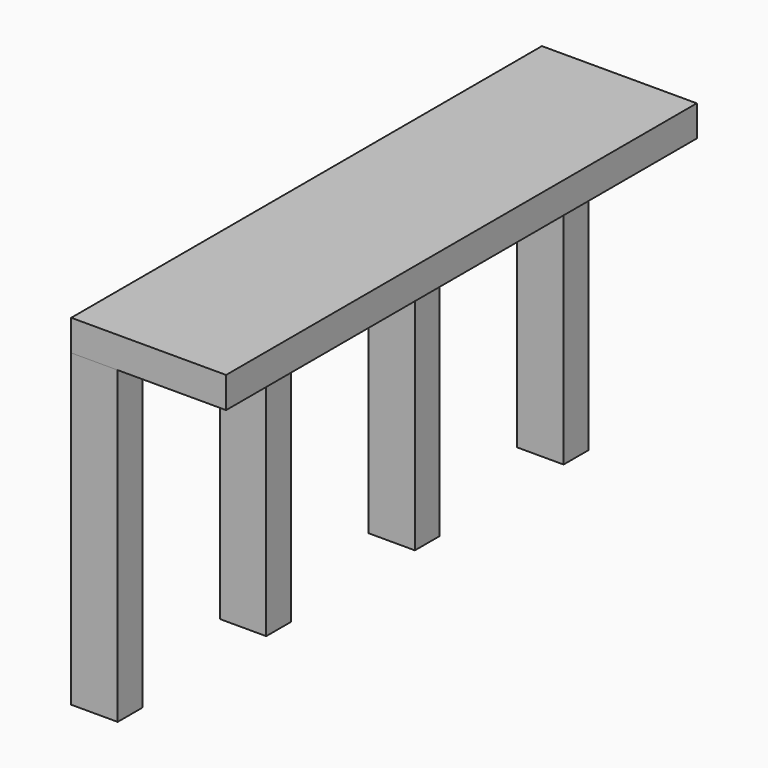
from build123d import *

# Parameters (mm, degrees)
F0_W     = 3
F0_H     = 2
F1_DEPTH = 20
F2_W     = 3
F2_H     = 2
F3_DEPTH = 2
F4_W     = 7.0251794532
F4_H     = 3.7774270773
F5_DEPTH = 25
F6_W     = 12.01007846
F6_H     = 2
F7_DEPTH = 25


with BuildPart() as f1:
    # F0 (on Top) → F1 (new body)
    with BuildSketch(Plane.XY):
        with Locations((1.5, 1)):
            Rectangle(F0_W, F0_H)
    extrude(amount=F1_DEPTH)


with BuildPart() as f1b:
    # F0 (on Top) → F1, piece 2 (new body)
    with BuildSketch(Plane.XY):
        with Locations((1.5, -11)):
            Rectangle(F0_W, F0_H)
    extrude(amount=F1_DEPTH)


with BuildPart() as f1c:
    # F0 (on Top) → F1, piece 3 (new body)
    with BuildSketch(Plane.XY):
        with Locations((1.5, -23)):
            Rectangle(F0_W, F0_H)
    extrude(amount=F1_DEPTH)


with BuildPart() as f1d:
    # F0 (on Top) → F1, piece 4 (new body)
    with BuildSketch(Plane.XY):
        with Locations((1.5, -35)):
            Rectangle(F0_W, F0_H)
    extrude(amount=F1_DEPTH)


with BuildPart() as f1e:
    # F0 (on Top) → F1, piece 5 (new body)
    with BuildSketch(Plane.XY):
        with Locations((1.5, -47)):
            Rectangle(F0_W, F0_H)
    extrude(amount=F1_DEPTH)


with BuildPart() as f1f:
    # F0 (on Top) → F1, piece 6 (new body)
    with BuildSketch(Plane.XY):
        with Locations((1.5, -59)):
            Rectangle(F0_W, F0_H)
    extrude(amount=F1_DEPTH)

    # F4 (on face) → F5 (cut)
    with BuildSketch(Plane.XY.offset(20)):
        with Locations((1.5459530987, -58.1112864614)):
            Rectangle(F4_W, F4_H)
    extrude(amount=-F5_DEPTH, mode=Mode.SUBTRACT)


with BuildPart() as f3:
    # F2 (on face) → F3 (new body)
    with BuildSketch(Plane.XY.offset(20)):
        with Locations((1.5, 1)):
            Rectangle(F2_W, F2_H)
        Polygon((10, 2), (3, 2), (3, 0), (0, 0), (0, -48), (10, -48), align=None)
    extrude(amount=F3_DEPTH)


with BuildPart() as f7_tool:
    # F6 (on face) → F7 (new body)
    with BuildSketch(Plane(origin=(0, 0, 0), x_dir=(0, -1, 0), z_dir=(-1, 0, 0))):
        with Locations((41.99496077, 21)):
            Rectangle(F6_W, F6_H)
        Polygon((48.0117946863, 22), (48, 22), (48, 20), (35.98992154, 20), (35.98992154, 0), (48.0117946863, 0), align=None)
    extrude(amount=-F7_DEPTH)


with BuildPart() as f1d_1:
    add(f1d.part)

    # F7: cut by f7_tool
    add(f7_tool.part, mode=Mode.SUBTRACT)


with BuildPart() as f1e_1:
    add(f1e.part)

    # F7: cut by f7_tool
    add(f7_tool.part, mode=Mode.SUBTRACT)


with BuildPart() as f3_1:
    add(f3.part)

    # F7: cut by f7_tool
    add(f7_tool.part, mode=Mode.SUBTRACT)


solid = Compound([f1.part, f1b.part, f1c.part, f1d_1.part, f3_1.part])
